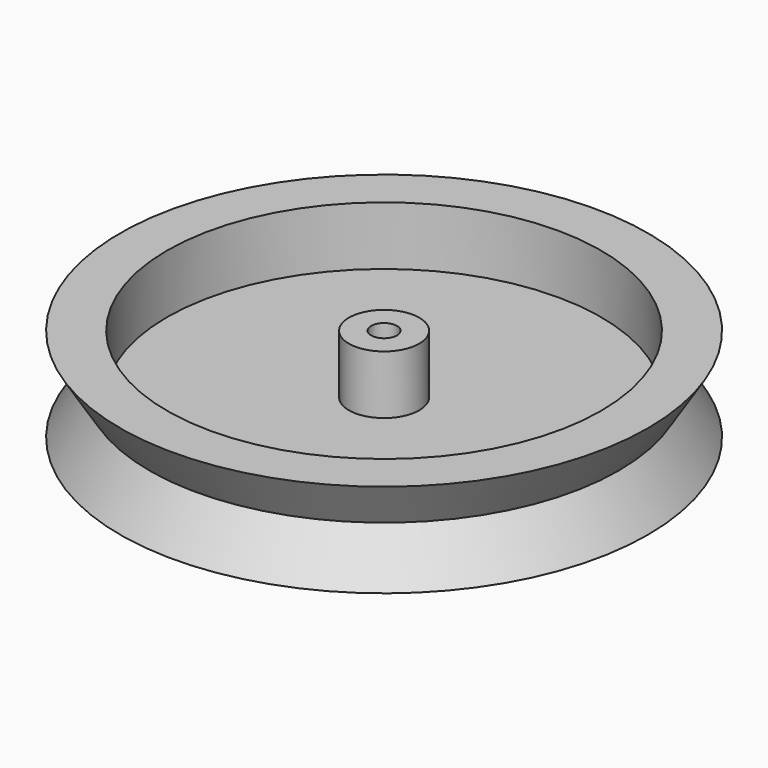
from build123d import *

# Parameters (mm, degrees)
F3_R     = 18.5
F4_DEPTH = 5
F5_R     = 3
F6_DEPTH = 5
F7_R     = 1.1
F8_DEPTH = 6


with BuildPart() as f2:
    # F1 (on Front) → F2 (revolve)
    with BuildSketch(Plane.XZ):
        Polygon((0, 8), (0, 0), (22.5, 0), (20, 4), (22.5, 8), align=None)
    revolve(axis=Axis((0, 0, 4), (0, 0, -1)))

    # F3 (on face) → F4 (cut)
    with BuildSketch(Plane.XY.offset(8)):
        Circle(F3_R)
    extrude(amount=-F4_DEPTH, mode=Mode.SUBTRACT)

    # F5 (on face) → F6 (join, through all)
    with BuildSketch(Plane.XY.offset(3)):
        Circle(F5_R)
    extrude(amount=F6_DEPTH)

    # F7 (on face) → F8 (cut)
    with BuildSketch(Plane.XY.offset(8)):
        Circle(F7_R)
    extrude(amount=-F8_DEPTH, mode=Mode.SUBTRACT)


solid = f2.part
